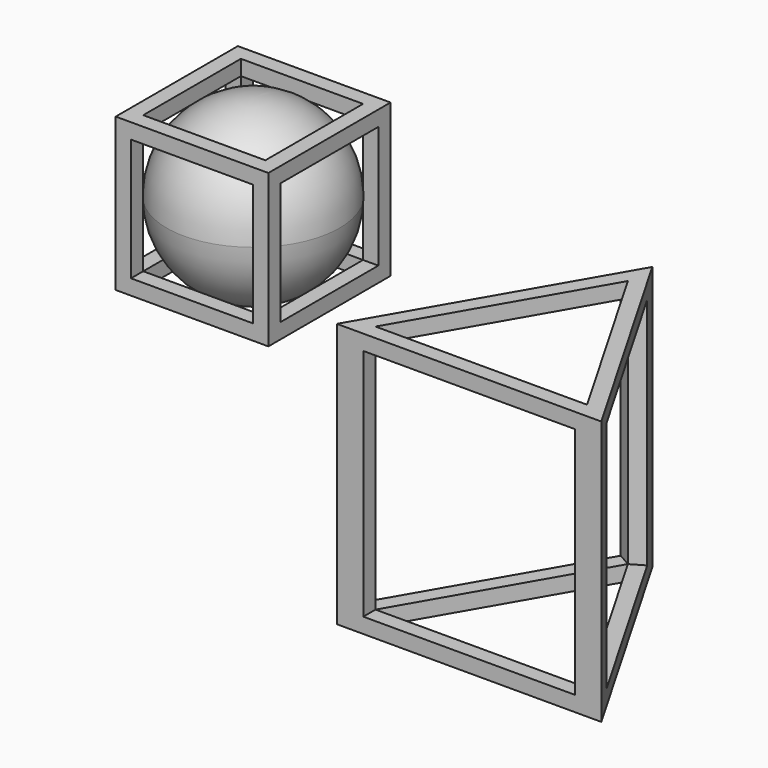
from build123d import *

# Parameters (mm, degrees)
F0_W      = 2.5
F0_H      = 2.5
F0_W_2    = 2
F0_H_2    = 2
F1_DEPTH  = 2.5
F2_W      = 2
F2_H      = 2
F3_DEPTH  = 25
F4_W      = 2
F4_H      = 2
F5_DEPTH  = 25
F7_DEPTH  = 4.33013
F12_W     = 3.4641016151
F12_H     = 3.83013
F13_DEPTH = 25
F14_W     = 3.4641016151
F14_H     = 3.83013
F15_DEPTH = 25
F16_W     = 3.4641016151
F16_H     = 3.83013
F17_DEPTH = 25


# Not quite as in the source:
# - a feature of the source that left no trace in its solid (it failed there, or was rolled back) is left out


with BuildPart() as f1:
    # F0 (on Top) → F1 (new body)
    with BuildSketch(Plane.XY):
        Rectangle(F0_W, F0_H)
        Rectangle(F0_W_2, F0_H_2, mode=Mode.SUBTRACT)
    extrude(amount=F1_DEPTH)

    # F2 (on face) → F3 (cut)
    with BuildSketch(Plane.XZ.offset(1.25)):
        with Locations((0, 1.25)):
            Rectangle(F2_W, F2_H)
    extrude(amount=-F3_DEPTH, mode=Mode.SUBTRACT)

    # F4 (on face) → F5 (cut)
    with BuildSketch(Plane.YZ.offset(1.25)):
        with Locations((0, 1.25)):
            Rectangle(F4_W, F4_H)
    extrude(amount=-F5_DEPTH, mode=Mode.SUBTRACT)


with BuildPart() as f7:
    # F6 (on Top) → F7 (new body)
    with BuildSketch(Plane.XY):
        Polygon((8.9044841006, -2.9603447206), (6.7394205912, -6.7103447206), (11.0695476101, -6.7103447206), align=None)
        Polygon((8.9044841006, -3.4603447206), (10.6365349082, -6.4603447206), (7.1724332931, -6.4603447206), align=None, mode=Mode.SUBTRACT)
    extrude(amount=F7_DEPTH)

    # F12 (on face) → F13 (cut)
    with BuildSketch(Plane(origin=(0, -6.4603447206, 0), x_dir=(-1, 0, 0), z_dir=(0, 1, 0))):
        with Locations((-8.9044841006, 2.165065)):
            Rectangle(F12_W, F12_H)
    extrude(amount=-F13_DEPTH, mode=Mode.SUBTRACT)

    # F14 (on face) → F15 (cut)
    with BuildSketch(Plane(origin=(5.1799898585, 2.9906685392, 0), x_dir=(0.5, -0.8660254038, 0), z_dir=(-0.8660254038, -0.5, 0))):
        with Locations((9.1810392918, 2.165065)):
            Rectangle(F14_W, F14_H)
    extrude(amount=-F15_DEPTH, mode=Mode.SUBTRACT)

    # F16 (on face) → F17 (cut)
    with BuildSketch(Plane(origin=(8.1767362924, -4.7208408995, 0), x_dir=(0.5, 0.8660254038, 0), z_dir=(0.8660254038, -0.5, 0))):
        with Locations((-0.2765551912, 2.165065)):
            Rectangle(F16_W, F16_H)
    extrude(amount=-F17_DEPTH, mode=Mode.SUBTRACT)


with BuildPart() as f11:
    # F10 (on Right) → F11 (revolve)
    with BuildSketch(Plane.YZ):
        with BuildLine():
            Line((0, 2.6642135624), (0, -0.1642135624))
            ThreePointArc((0, -0.1642135624), (1, 0.25), (1.4142135624, 1.25))
            ThreePointArc((1.4142135624, 1.25), (1, 2.25), (0, 2.6642135624))
        make_face()
    revolve(axis=Axis((0, 0, 1.25), (0, 0, 1)))


solid = Compound([f1.part, f7.part, f11.part])
